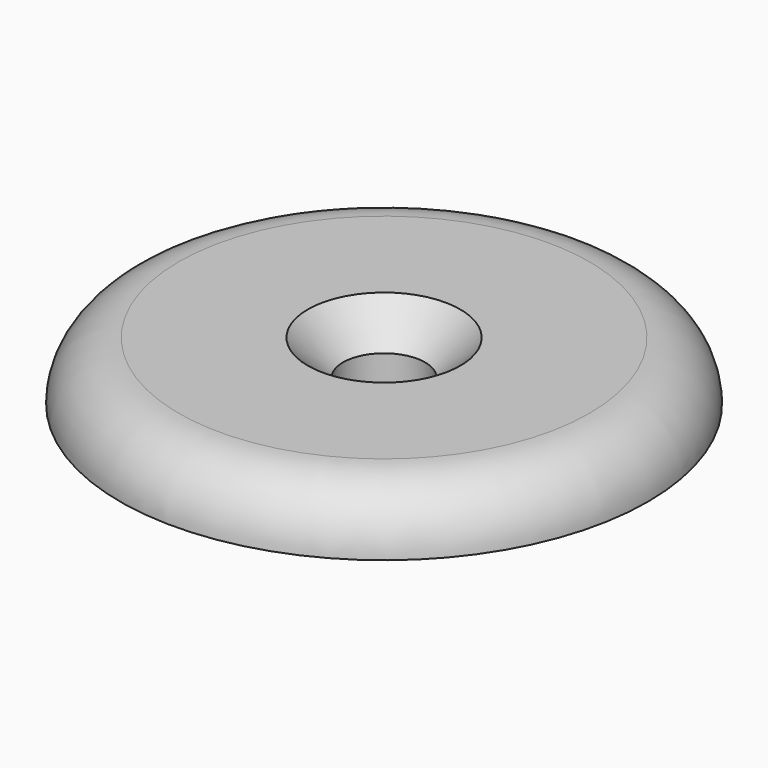
from build123d import *

# Parameters (mm, degrees)
F0_R           = 11.25
F1_DEPTH       = 2.5
F2_R           = 2.49999
F4_R           = 4.05
F5_DEPTH       = 2.5
F6_D           = 3.5
F6_DEPTH       = 7
F6_CSINK_D     = 6.5
F6_CSINK_ANGLE = 90
F6_TIP         = 1.0515060833


# Not quite as in the source:
# - a fillet or chamfer is up to 0.001 mm smaller than in the source, because OpenCascade refuses the exact size


with BuildPart() as f1:
    # F0 (on Top) → F1 (new body)
    with BuildSketch(Plane.XY):
        Circle(F0_R)
    extrude(amount=F1_DEPTH)

    # F2 (radius 2.5 in the source; OpenCascade refuses exactly that, so slightly less here)
    f2_edges = [f1.edges().sort_by_distance(p)[0] for p in [
        (-11.25, 0, 2.5),
    ]]
    fillet(f2_edges, radius=F2_R)

    # F4 (on face) → F5 (join)
    with BuildSketch(Plane(origin=(0, 0, 0), x_dir=(1, 0, 0), z_dir=(0, 0, -1))):
        Circle(F4_R)
    extrude(amount=F5_DEPTH)

    # F6
    with Locations(Plane.XY.offset(2.5)):
        with Locations((0, 0)):
            CounterSinkHole(F6_D / 2, F6_CSINK_D / 2, depth=F6_DEPTH, counter_sink_angle=F6_CSINK_ANGLE)
            with Locations((0, 0, -(F6_DEPTH + F6_TIP / 2))):  # 118° drill point
                Cone(0, F6_D / 2, F6_TIP, mode=Mode.SUBTRACT)


solid = f1.part
